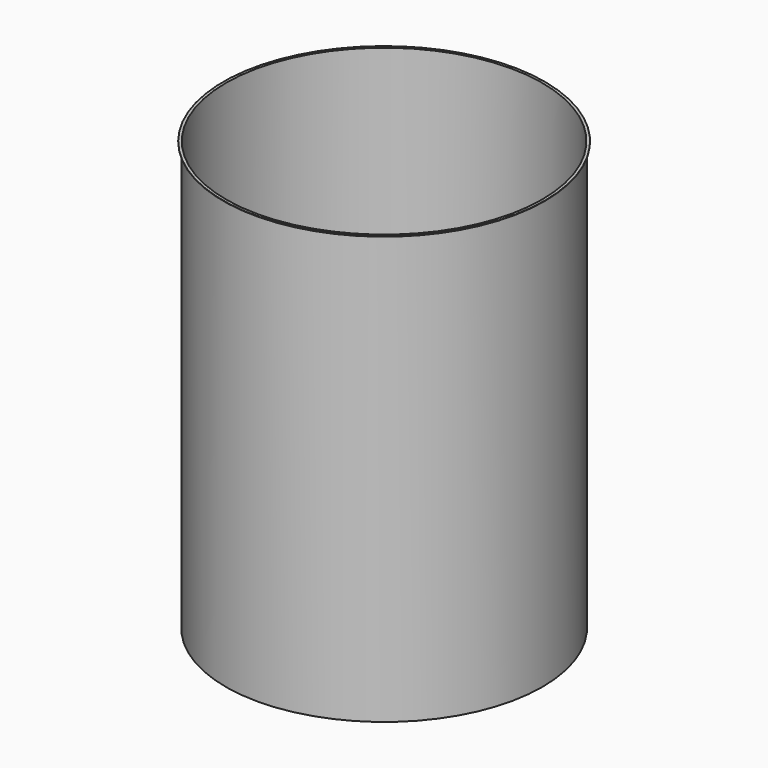
from build123d import *

# Parameters (mm, degrees)
F0_R     = 5029.2
F0_R_2   = 5016.5
F1_DEPTH = 13615.416
F2_R     = 5016.5
F3_DEPTH = 6.35
F4_R     = 5105.4
F4_R_2   = 5029.2
F5_DEPTH = 12.7
F6_R     = 5041.9
F6_R_2   = 5029.2
F7_DEPTH = 50.8


with BuildPart() as f1:
    # F0 (on Top) → F1 (new body)
    with BuildSketch(Plane.XY):
        Circle(F0_R)
        Circle(F0_R_2, mode=Mode.SUBTRACT)
    extrude(amount=F1_DEPTH)

    # F4 (on face) → F5 (join)
    with BuildSketch(Plane.XY.offset(13615.416)):
        Circle(F4_R)
        Circle(F4_R_2, mode=Mode.SUBTRACT)
    extrude(amount=-F5_DEPTH)

    # F6 (on face) → F7 (join)
    with BuildSketch(Plane(origin=(0, 0, 13602.716), x_dir=(1, 0, 0), z_dir=(0, 0, -1))):
        Circle(F6_R)
        Circle(F6_R_2, mode=Mode.SUBTRACT)
    extrude(amount=F7_DEPTH)


with BuildPart() as f3:
    # F2 (on face) → F3 (new body)
    with BuildSketch(Plane(origin=(0, 0, 0), x_dir=(1, 0, 0), z_dir=(0, 0, -1))):
        Circle(F2_R)
    extrude(amount=F3_DEPTH)


with BuildPart() as f1_1:
    add(f1.part)

    # F8: union F3
    add(f3.part)


solid = f1_1.part
